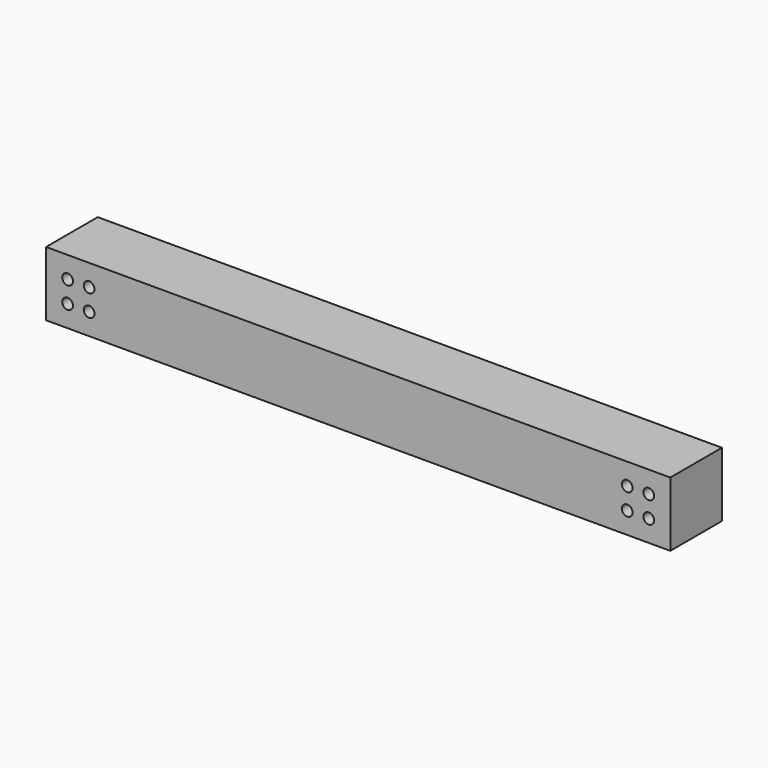
from build123d import *

# Parameters (mm, degrees)
F0_W     = 290
F0_H     = 30
F1_DEPTH = 15
F3_D     = 5


# Not quite as in the source:
# - a feature names something its author has since deleted; it is built from what else it names


with BuildPart() as f1:
    # F0 (on Front) → F1 (new body, symmetric)
    with BuildSketch(Plane.XZ):
        Rectangle(F0_W, F0_H)
    extrude(amount=F1_DEPTH, both=True)

    # F3 (through all)
    with Locations(Plane.XZ.offset(15)):
        with Locations((-135, 5), (-135, -5), (-125, 5), (-125, -5), (125, 5), (125, -5), (135, 5), (135, -5)):
            Hole(F3_D / 2)


solid = f1.part
